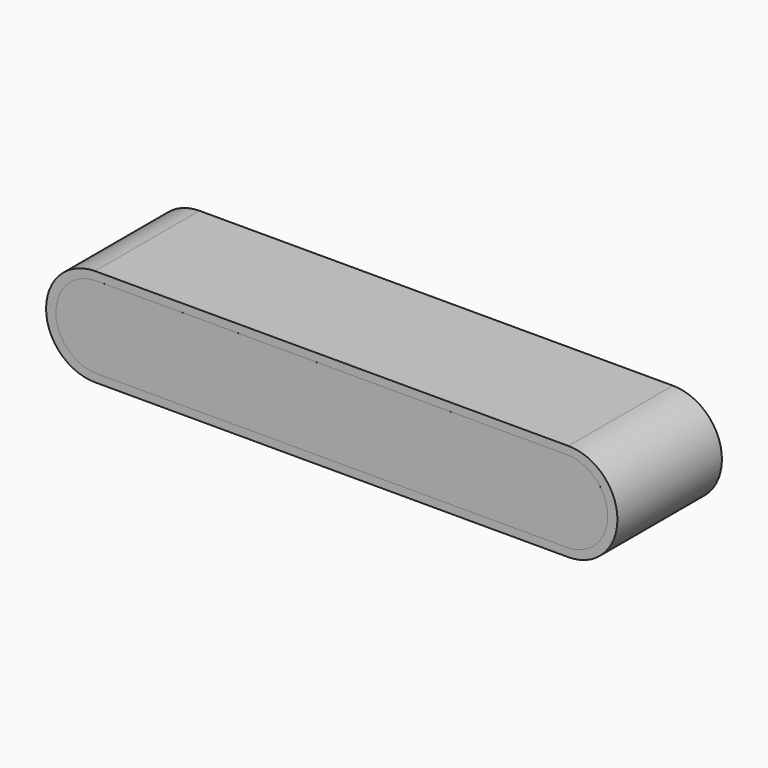
from build123d import *

# Parameters (mm, degrees)
F0_W     = 175
F0_H     = 40
F1_DEPTH = 15
F3_DEPTH = 50.8
F5_DEPTH = 0.001


# Not quite as in the source:
# - a feature names something its author has since deleted; it is built from what else it names


with BuildPart() as f1:
    # F0 (on Top) → F1 (new body, symmetric)
    with BuildSketch(Plane.XY):
        Rectangle(F0_W, F0_H)
    extrude(amount=F1_DEPTH, both=True)

    # F2 (on face) → F3 (cut)
    with BuildSketch(Plane.XZ.offset(20)):
        with BuildLine():
            ThreePointArc((-87.5, 0), (-83.1066017178, 10.6066017178), (-72.5, 15))
            Line((-72.5, 15), (-87.5, 15))
            Line((-87.5, 15), (-87.5, 0))
        make_face()
        with BuildLine():
            Line((-87.5, -15), (-72.5, -15))
            ThreePointArc((-72.5, -15), (-83.1066017178, -10.6066017178), (-87.5, 0))
            Line((-87.5, 0), (-87.5, -15))
        make_face()
        with BuildLine():
            ThreePointArc((87.5, 0), (83.1066017178, -10.6066017178), (72.5, -15))
            Line((72.5, -15), (87.5, -15))
            Line((87.5, -15), (87.5, 0))
        make_face()
        with BuildLine():
            Line((87.5, 15), (72.5, 15))
            ThreePointArc((72.5, 15), (83.1066017178, 10.6066017178), (87.5, 0))
            Line((87.5, 0), (87.5, 15))
        make_face()
    extrude(amount=-F3_DEPTH, mode=Mode.SUBTRACT)

    # F4 (on face) → F5 (join)
    with BuildSketch(Plane.XZ.offset(20)):
        with BuildLine():
            Line((72, 12.5), (-72, 12.5))
            ThreePointArc((-72, 12.5), (-84.5, 0), (-72, -12.5))
            Line((-72, -12.5), (0, -12.5))
            Line((0, -12.5), (72, -12.5))
            ThreePointArc((72, -12.5), (84.5, 0), (72, 12.5))
        make_face()
    extrude(amount=F5_DEPTH)


solid = f1.part
